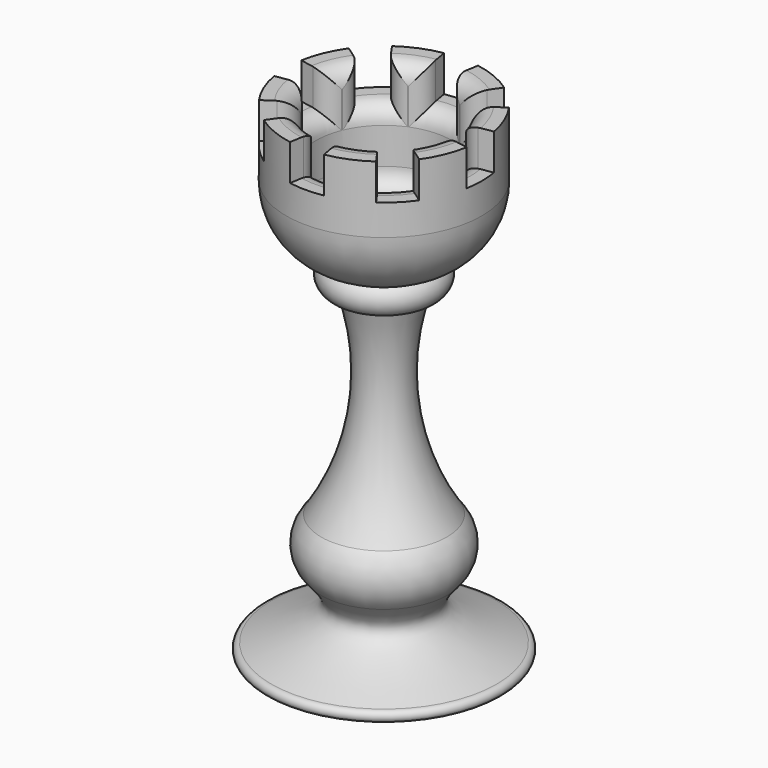
from build123d import *

# Parameters (mm, degrees)
F2_R     = 6.8817481914
F3_DEPTH = 9.525
F4_R     = 4.7625
F5_DEPTH = 7.62
F7_DEPTH = 2.54
F9_R     = 1.27


# Not quite as in the source:
# - a fillet or chamfer that OpenCascade refuses, or shapes differently, is made with other operations: its cross-section is extruded or revolved along the edge and cut away or added


with BuildPart() as f1:
    # F0 (on Front) → F1 (revolve)
    with BuildSketch(Plane.XZ):
        with BuildLine():
            Line((3.4089614412, 24.5809284006), (0, 24.5809284006))
            Line((0, 24.5809284006), (0, 0))
            Line((0, 0), (7.9375, 0))
            ThreePointArc((7.9375, 0), (8.3142796152, 0.3767796152), (7.9375, 0.7535592304))
            add(Edge.make_bspline(
                [(4.4289799407, 5.0970371813), (3.8652116037, 4.447307109), (2.4266767475, 2.7894286959), (5.8536021882, 1.5234158797), (7.9375, 0.7535592304)],
                knots=[0, 0, 0, 0, 0.3919045372, 1, 1, 1, 1], degree=3))
            ThreePointArc((4.4289799407, 5.0970371813), (5.1574363772, 6.9059464149), (4.4289799407, 8.7148556486))
            ThreePointArc((4.4289799407, 8.7148556486), (1.9305085977, 15.5362857998), (2.6656309819, 22.7635856718))
            Line((2.6656309819, 22.7635856718), (3.4089614412, 22.7635856718))
            ThreePointArc((3.4089614412, 22.7635856718), (3.8588998931, 23.6722570362), (3.4089614412, 24.5809284006))
        make_face()
    revolve(axis=Axis((0, 0, 12.2904642003), (0, 0, -1)))

    # F2 (on face) → F3 (join)
    with BuildSketch(Plane.XY.offset(24.5809284006)):
        Circle(F2_R)
    extrude(amount=F3_DEPTH)

    # F4 (on face) → F5 (cut)
    with BuildSketch(Plane.XY.offset(34.1059284006)):
        Circle(F4_R)
    extrude(amount=-F5_DEPTH, mode=Mode.SUBTRACT)

    # F6 (on face) → F7 (cut)
    with BuildSketch(Plane.XY.offset(34.1059284006)):
        with BuildLine():
            Line((6.7771989732, 1.1950030326), (4.6901469237, 0.8269994461))
            ThreePointArc((4.6901469237, 0.8269994461), (4.7443772497, 0.4150792248), (4.7625, 0))
            ThreePointArc((4.7625, 0), (4.7443772497, -0.4150792248), (4.6901469237, -0.8269994461))
            Line((4.6901469237, -0.8269994461), (6.7771989732, -1.1950030326))
            ThreePointArc((6.7771989732, -1.1950030326), (6.8555610619, -0.599783875), (6.8817481914, 0))
            ThreePointArc((6.8817481914, 0), (6.8555610619, 0.599783875), (6.7771989732, 1.1950030326))
        make_face()
        with BuildLine():
            ThreePointArc((2.7316577781, 3.9012116109), (3.3675960454, 3.3675960454), (3.9012116109, 2.7316577781))
            Line((3.9012116109, 2.7316577781), (5.6371980993, 3.9472086035))
            ThreePointArc((5.6371980993, 3.9472086035), (4.8661308126, 4.8661308126), (3.9472086035, 5.6371980993))
            Line((3.9472086035, 5.6371980993), (2.7316577781, 3.9012116109))
        make_face()
        with BuildLine():
            ThreePointArc((-0.8269994461, 4.6901469237), (0, 4.7625), (0.8269994461, 4.6901469237))
            Line((0.8269994461, 4.6901469237), (1.1950030326, 6.7771989732))
            ThreePointArc((1.1950030326, 6.7771989732), (0, 6.8817481914), (-1.1950030326, 6.7771989732))
            Line((-1.1950030326, 6.7771989732), (-0.8269994461, 4.6901469237))
        make_face()
        with BuildLine():
            ThreePointArc((-3.9012116109, 2.7316577781), (-3.3675960454, 3.3675960454), (-2.7316577781, 3.9012116109))
            Line((-2.7316577781, 3.9012116109), (-3.9472086035, 5.6371980993))
            ThreePointArc((-3.9472086035, 5.6371980993), (-4.8661308126, 4.8661308126), (-5.6371980993, 3.9472086035))
            Line((-5.6371980993, 3.9472086035), (-3.9012116109, 2.7316577781))
        make_face()
        with BuildLine():
            ThreePointArc((-4.6901469237, -0.8269994461), (-4.7625, 0), (-4.6901469237, 0.8269994461))
            Line((-4.6901469237, 0.8269994461), (-6.7771989732, 1.1950030326))
            ThreePointArc((-6.7771989732, 1.1950030326), (-6.8817481914, 0), (-6.7771989732, -1.1950030326))
            Line((-6.7771989732, -1.1950030326), (-4.6901469237, -0.8269994461))
        make_face()
        with BuildLine():
            Line((-3.9472086035, -5.6371980993), (-2.7316577781, -3.9012116109))
            ThreePointArc((-2.7316577781, -3.9012116109), (-3.3675960454, -3.3675960454), (-3.9012116109, -2.7316577781))
            Line((-3.9012116109, -2.7316577781), (-5.6371980993, -3.9472086035))
            ThreePointArc((-5.6371980993, -3.9472086035), (-4.8661308126, -4.8661308126), (-3.9472086035, -5.6371980993))
        make_face()
        with BuildLine():
            Line((1.1950030326, -6.7771989732), (0.8269994461, -4.6901469237))
            ThreePointArc((0.8269994461, -4.6901469237), (0, -4.7625), (-0.8269994461, -4.6901469237))
            Line((-0.8269994461, -4.6901469237), (-1.1950030326, -6.7771989732))
            ThreePointArc((-1.1950030326, -6.7771989732), (0, -6.8817481914), (1.1950030326, -6.7771989732))
        make_face()
        with BuildLine():
            Line((5.6371980993, -3.9472086035), (3.9012116109, -2.7316577781))
            ThreePointArc((3.9012116109, -2.7316577781), (3.3675960454, -3.3675960454), (2.7316577781, -3.9012116109))
            Line((2.7316577781, -3.9012116109), (3.9472086035, -5.6371980993))
            ThreePointArc((3.9472086035, -5.6371980993), (4.8661308126, -4.8661308126), (5.6371980993, -3.9472086035))
        make_face()
    extrude(amount=-F7_DEPTH, mode=Mode.SUBTRACT)

    # F8: fillet of radius 5.08 on 1 edges, made by hand

    # F8_s1 → F8_t2 (revolve, cut)
    with BuildSketch(Plane.XZ):
        with BuildLine():
            ThreePointArc((6.8817481914, 29.3999807524), (5.9230976857, 26.4299843979), (3.4089614412, 24.5809284006))
            Line((3.4089614412, 24.5809284006), (6.8817481914, 24.5809284006))
            Line((6.8817481914, 24.5809284006), (6.8817481914, 29.3999807524))
        make_face()
    revolve(axis=Axis((0, 0, 24.5809284006), (0, 0, 1)), mode=Mode.SUBTRACT)

    # F9
    f9_edges = [f1.edges().sort_by_distance(p)[0] for p in [
        (4.744377, 0.415079, 31.565928),
        (4.690147, 0.826999, 32.835928),
        (4.399976, 1.82253, 34.105928),
        (3.901212, 2.731658, 32.835928),
        (3.367596, 3.367596, 31.565928),
        (2.731658, 3.901212, 32.835928),
        (1.82253, 4.399976, 34.105928),
        (0.826999, 4.690147, 32.835928),
        (0, 4.7625, 31.565928),
        (-0.826999, 4.690147, 32.835928),
        (-1.82253, 4.399976, 34.105928),
        (-2.731658, 3.901212, 32.835928),
        (-3.367596, 3.367596, 31.565928),
        (-3.901212, 2.731658, 32.835928),
        (-4.399976, 1.82253, 34.105928),
        (-4.690147, 0.826999, 32.835928),
        (-4.7625, 0, 31.565928),
        (-4.690147, -0.826999, 32.835928),
        (-4.399976, -1.82253, 34.105928),
        (-3.901212, -2.731658, 32.835928),
        (-3.367596, -3.367596, 31.565928),
        (-2.731658, -3.901212, 32.835928),
        (-1.82253, -4.399976, 34.105928),
        (-0.826999, -4.690147, 32.835928),
        (0, -4.7625, 31.565928),
        (0.826999, -4.690147, 32.835928),
        (1.82253, -4.399976, 34.105928),
        (2.731658, -3.901212, 32.835928),
        (3.367596, -3.367596, 31.565928),
        (3.901212, -2.731658, 32.835928),
        (4.399976, -1.82253, 34.105928),
        (4.690147, -0.826999, 32.835928),
        (4.744377, -0.415079, 31.565928),
        (4.7625, 0, 29.025928),
        (-4.7625, 0, 26.485928),
    ]]
    fillet(f9_edges, radius=F9_R)


solid = f1.part
